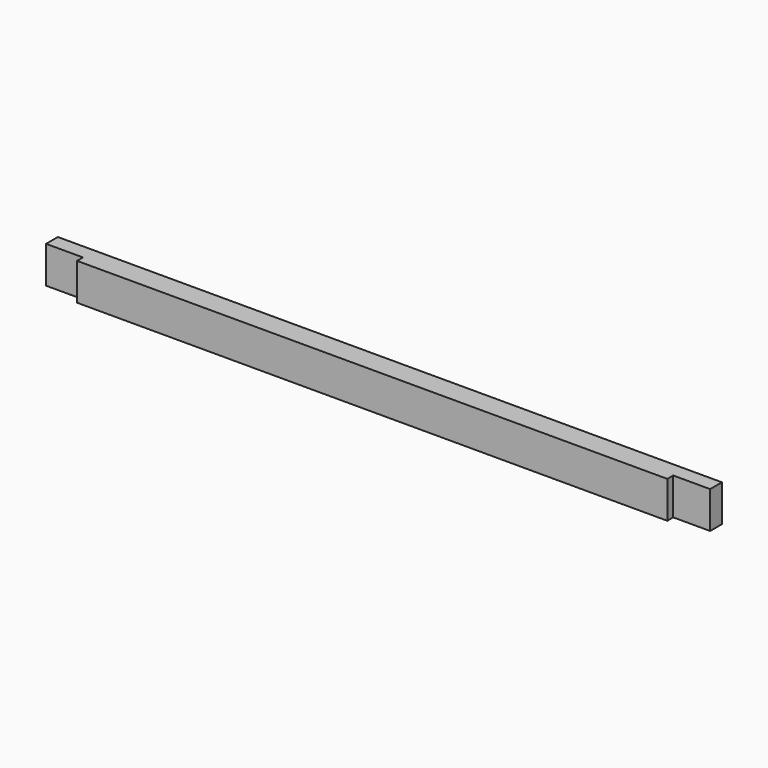
from build123d import *

# Parameters (mm, degrees)
F1_W     = 60
F1_H     = 100
F2_DEPTH = 800
F3_W     = 40
F3_H     = 100
F4_DEPTH = 100


# Not quite as in the source:
# - a pattern or mirror of a feature is missing from the dataset's text; its kind, count and spacing are read off the source's solid


with BuildPart() as f2:
    # F1 (on Right) → F2 (new body, symmetric)
    with BuildSketch(Plane.YZ):
        Rectangle(F1_W, F1_H)
    extrude(amount=F2_DEPTH, both=True)

    # F3 (on face) → F4 (join)
    with BuildSketch(Plane(origin=(-800, 0, 0), x_dir=(0, -1, 0), z_dir=(-1, 0, 0))):
        with Locations((-10, 0)):
            Rectangle(F3_W, F3_H)
    f4 = extrude(amount=F4_DEPTH)

    # F4_copies: F4 across plane
    add(f4.mirror(Plane(origin=(0, 0, 0), x_dir=(0, 0, 1), z_dir=(1, 0, 0))))


solid = f2.part
